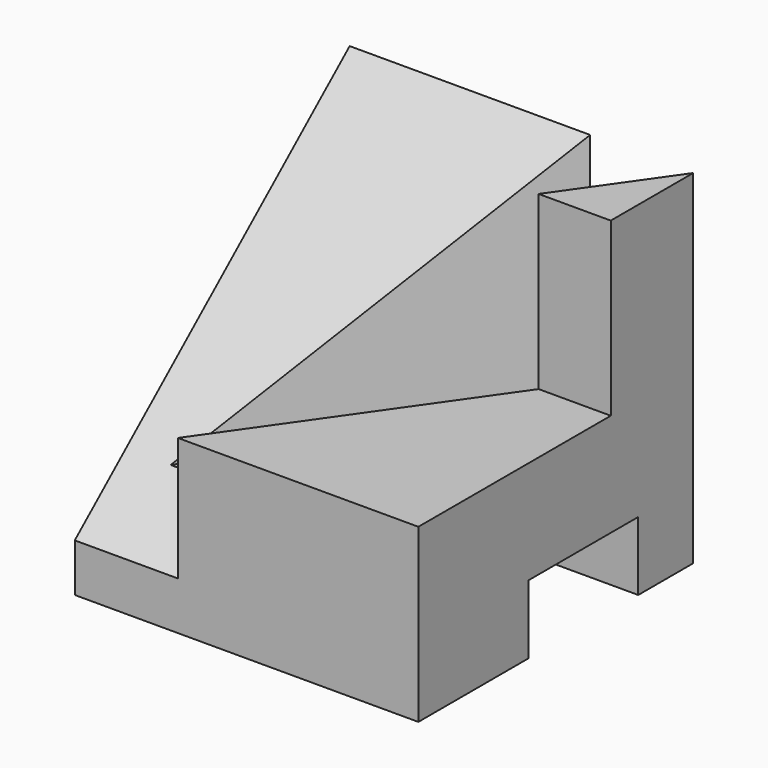
from build123d import *

# Parameters (mm, degrees)
F0_W      = 50
F0_H      = 50
F1_DEPTH  = 50
F2_W      = 20
F2_H      = 10
F4_DEPTH  = 30
F7_DEPTH  = 25
F9_DEPTH  = 35
F11_REACH = 115.9479483752


with BuildPart() as f1:
    # F0 (on Top) → F1 (new body)
    with BuildSketch(Plane.XY):
        with Locations((-3.8959849626, 9.4470265827)):
            Rectangle(F0_W, F0_H)
    extrude(amount=F1_DEPTH)

    # F2 (on face) → F4 (cut, through all)
    with BuildSketch(Plane.YZ.offset(21.1040150374)):
        with Locations((14.4470265827, 5)):
            Rectangle(F2_W, F2_H)
    extrude(amount=-F4_DEPTH, mode=Mode.SUBTRACT)

    # F5 (on face) → F7 (cut, through all)
    with BuildSketch(Plane.XY.offset(50)):
        Polygon((21.1040150374, 19.4470265827), (10.6040150374, 19.4470265827), (-13.8959849626, -15.5529734173), (21.1040150374, -15.5529734173), align=None)
    extrude(amount=-F7_DEPTH, mode=Mode.SUBTRACT)

    # F5 (on face) → F9 (cut, through all)
    with BuildSketch(Plane.XY.offset(50)):
        Polygon((10.6040150374, 19.4470265827), (21.1040150374, 34.4470265827), (6.1040150374, 34.4470265827), (-28.8959849626, -15.5529734173), (-13.8959849626, -15.5529734173), align=None)
    extrude(amount=-F9_DEPTH, mode=Mode.SUBTRACT)

    f11_end = Plane(origin=(8.8540150374, 16.9470265827, 27.5), x_dir=(-0.5734623444, -0.8192319205, 0), z_dir=(-0.8192319205, 0.5734623444, 0))
    # F10 (on face) → F11 (cut, up to a plane its end follows)
    with BuildSketch(Plane(origin=(-28.8959849626, 0, 0), x_dir=(0, -1, 0), z_dir=(-1, 0, 0))):
        Polygon((15.5529734173, 7), (15.5529734173, 50), (-34.4470265827, 50), align=None)
    f11_long = extrude(amount=-F11_REACH, mode=Mode.PRIVATE)
    add(split(f11_long, bisect_by=f11_end, keep=Keep.TOP, mode=Mode.PRIVATE), mode=Mode.SUBTRACT)


solid = f1.part
